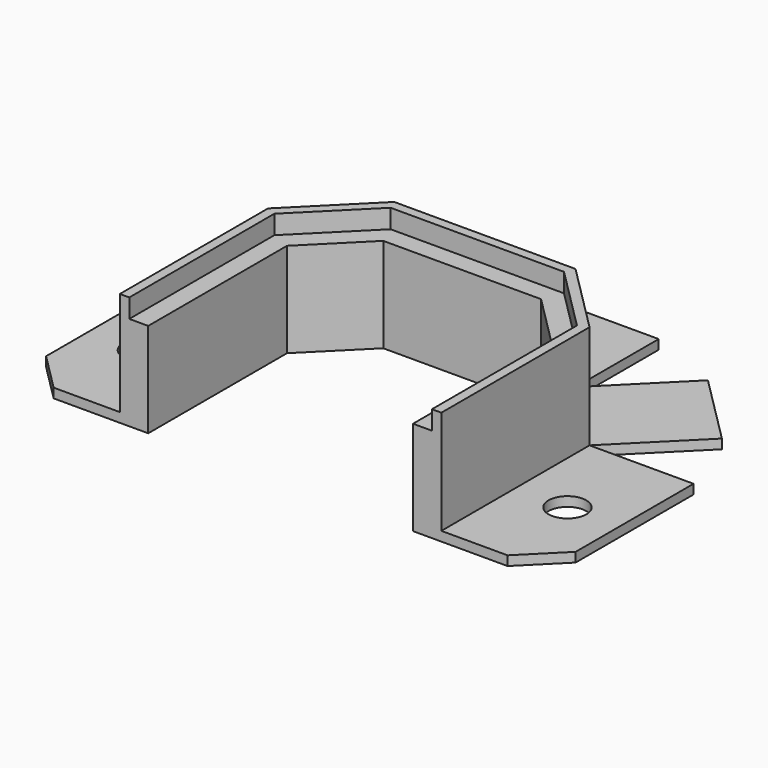
from build123d import *

# Parameters (mm, degrees)
F4_D     = 12.7
F4_DEPTH = 12.7
F4_TIP   = 3.8154649308
F6_DEPTH = 3.176
F7_SIZE  = 12.7


# Not quite as in the source:
# - a feature names something its author has since deleted; it is built from what else it names


with BuildPart() as f2:
    # F2: sweep along a path in F1
    with BuildLine(Plane.XY) as f2_path:
        Line((-44.45, 0), (-44.45, 58.2394877579))
        Line((-44.45, 58.2394877579), (-26.4894877579, 76.2))
        Line((-26.4894877579, 76.2), (26.4894877579, 76.2))
        Line((26.4894877579, 76.2), (44.45, 58.2394877579))
        Line((44.45, 58.2394877579), (44.45, 0))
    # F0 (on Front) → F2 (sweep)
    with BuildSketch(Plane.XZ):
        Polygon((-50.8, 38.1), (-53.975, 38.1), (-53.975, 3.175), (-88.9, 3.175), (-88.9, 0), (-53.975, 0), (-50.8, 0), (-50.8, 3.175), (-50.8, 31.75), align=None)
        Polygon((-44.45, 31.75), (-50.8, 31.75), (-50.8, 3.175), (-50.8, 0), (-44.45, 0), align=None)
    sweep(path=f2_path.line, transition=Transition.RIGHT)

    # F4
    with Locations(Plane.XY.offset(3.175)):
        with Locations((-71.4375, 31.0896), (71.4375, 31.0896), (0, 103.1875)):
            Hole(F4_D / 2, depth=F4_DEPTH)
            with Locations((0, 0, -(F4_DEPTH + F4_TIP / 2))):  # 118° drill point
                Cone(0, F4_D / 2, F4_TIP, mode=Mode.SUBTRACT)

    # F5 (on face) → F6 (cut, through all)
    with BuildSketch(Plane.XY.offset(3.175)):
        Polygon((-88.9, 62.1848719395), (-53.975, 62.1848719395), (-78.6707043329, 86.8805762724), (-88.9, 76.6512806053), align=None)
        Polygon((-55.1305762724, 110.4207043329), (-30.4348719395, 85.725), (-30.4348719395, 120.65), (-44.9012806053, 120.65), align=None)
        Polygon((30.4348719395, 120.65), (30.4348719395, 85.725), (55.1305762724, 110.4207043329), (44.9012806053, 120.65), align=None)
        Polygon((78.6707043329, 86.8805762724), (53.975, 62.1848719395), (88.9, 62.1848719395), (88.9, 76.6512806053), align=None)
    extrude(amount=-F6_DEPTH, mode=Mode.SUBTRACT)

    # F7
    f7_edges = [f2.edges().sort_by_distance(p)[0] for p in [
        (-88.9, 0, 1.5875),
        (88.9, 0, 1.5875),
    ]]
    chamfer(f7_edges, length=F7_SIZE)


solid = f2.part
